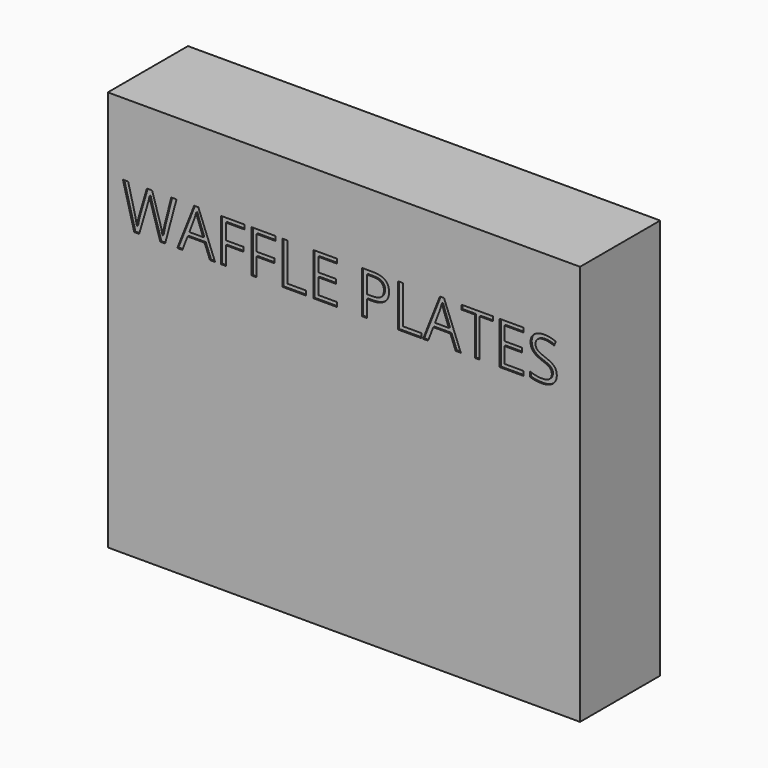
from build123d import *

# Parameters (mm, degrees)
F0_W         = 330
F0_H         = 70
F1_DEPTH     = 280
F2_TEXT_SIZE = 41.6666666667
F3_DEPTH     = 1


# Not quite as in the source:
# - Text() gives the source's letters only with a copy of the font that has no kerning and outlines rounded to 1/6400 em; it was checked with that copy


with BuildPart() as f1:
    # F0 (on Top) → F1 (new body)
    with BuildSketch(Plane.XY):
        Rectangle(F0_W, F0_H)
    extrude(amount=F1_DEPTH)

    # F2 (on face) → F3 (cut)
    with BuildSketch(Plane.XZ.offset(35)):
        with Locations((-155, 200)):
            Text('WAFFLE PLATES', F2_TEXT_SIZE, font='Open Sans', text_align=(TextAlign.LEFT, TextAlign.BOTTOM))
    extrude(amount=-F3_DEPTH, mode=Mode.SUBTRACT)


solid = f1.part
